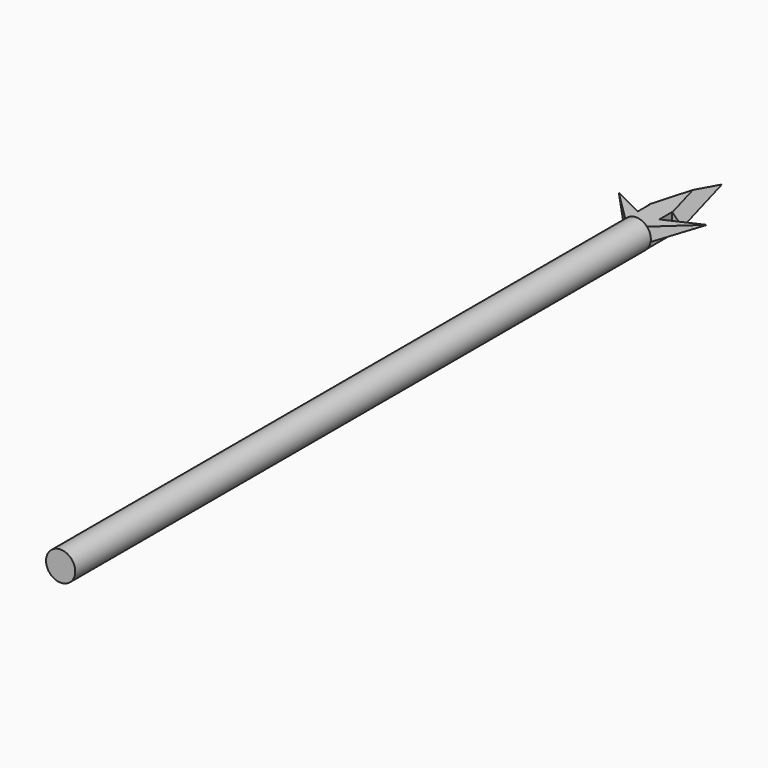
from build123d import *

# Parameters (mm, degrees)
F0_R          = 3.81
F1_DEPTH      = 187.71276
F3_DEPTH      = 2.54
F3_DEPTH_BACK = 2.59802
F4_SIZE       = 5.08
F5_T4_DEPTH   = 56.2135595652
F5_T10_DEPTH  = 56.3150595014
F5_T17_DEPTH  = 56.2135595652
F5_T21_DEPTH  = 56.3150595014
F6_T4_DEPTH   = 35.2698827679
F6_T9_DEPTH   = 36.002021323


# Not quite as in the source:
# - a fillet or chamfer that OpenCascade refuses, or shapes differently, is made with other operations: its cross-section is extruded or revolved along the edge and cut away or added


with BuildPart() as f1:
    # F0 (on Front) → F1 (new body)
    with BuildSketch(Plane.XZ):
        Circle(F0_R)
    extrude(amount=-F1_DEPTH)


with BuildPart() as f3:
    # F2 (on Top) → F3 (new body, two sides)
    with BuildSketch(Plane.XY) as f3_sk:
        Polygon((-2.8854149859, 191.8134321757), (-2.8854149859, 187.7436647788), (2.7261148207, 187.7214848121), (2.7261148207, 191.8280913989), (2.7261148207, 195.9346979856), (8.1146247685, 195.9346979856), (0, 224.9049544334), (-8.3053142529, 195.8831995726), (-2.8854149859, 195.8831995726), align=None)
        Polygon((-11.071106419, 195.8831995726), (-2.8854149859, 187.7436647788), (-2.8854149859, 191.8134321757), align=None)
        Polygon((2.7261148207, 191.8280913989), (2.7261148207, 187.7214848121), (11.7052067071, 195.9349513054), align=None)
    extrude(amount=F3_DEPTH)
    extrude(f3_sk.sketch, amount=-F3_DEPTH_BACK)

    # F4
    f4_edges = [f3.edges().sort_by_distance(p)[0] for p in [
        (4.057312, 210.419826, -2.59802),
        (-4.152657, 210.394077, -2.59802),
    ]]
    chamfer(f4_edges, length=F4_SIZE)

    # F5: chamfer of 5.08 on 2 edges, made by hand


with BuildPart() as f5_tool2:
    # F5_s3 → F5_t4 (new body)
    with BuildSketch(Plane(origin=(-46.7750694582, 166.9930275555, 0), x_dir=(0, 0, 1), z_dir=(-0.2697209417, 0.9629385305, 0))):
        with BuildLine():
            Line((-2.6836840979, 60.8052602015), (2.6836840979, 55.4378920056))
            Line((2.6836840979, 55.4378920056), (2.7852840979, 55.4378920056))
            ThreePointArc((2.7852840979, 55.4378920056), (2.6416, 58.0497340546), (2.6416, 60.6615761036))
            Line((2.6416, 60.6615761036), (2.54, 60.7631761036))
            ThreePointArc((2.54, 60.7631761036), (-0.071842049, 60.7631761036), (-2.6836840979, 60.9068602015))
            Line((-2.6836840979, 60.9068602015), (-2.6836840979, 60.8052602015))
        make_face()
    extrude(amount=F5_T4_DEPTH)

    split(bisect_by=Plane.XZ.offset(-195.9346979856), keep=Keep.BOTTOM)

    split(bisect_by=Plane(origin=(-59.4902437107, 17.0246482808, 0), x_dir=(0, 0, 1), z_dir=(0.9614067403, -0.275131023, 0)), keep=Keep.TOP)


with BuildPart() as f3_1:
    add(f3.part)

    # F5_t1: cut F5_tool2
    add(f5_tool2.part, mode=Mode.SUBTRACT)


with BuildPart() as f5_tool8:
    # F5_s9 → F5_t10 (new body)
    with BuildSketch(Plane(origin=(63.0845965483, 220.4402676135, 0), x_dir=(0, 0, 1), z_dir=(-0.275131023, -0.9614067403, 0))):
        with BuildLine():
            Line((2.6836840979, 56.6546460819), (-2.6836840979, 62.0220142778))
            Line((-2.6836840979, 62.0220142778), (-2.6836840979, 62.1236142778))
            ThreePointArc((-2.6836840979, 62.1236142778), (-0.071842049, 61.9799301798), (2.54, 61.9799301798))
            Line((2.54, 61.9799301798), (2.6416, 61.8783301798))
            ThreePointArc((2.6416, 61.8783301798), (2.6416, 59.2664881309), (2.7852840979, 56.6546460819))
            Line((2.7852840979, 56.6546460819), (2.6836840979, 56.6546460819))
        make_face()
    extrude(amount=F5_T10_DEPTH)

    split(bisect_by=Plane.XZ.offset(-195.8831995726), keep=Keep.BOTTOM)

    split(bisect_by=Plane(origin=(58.4133689537, 16.3616974319, 0), x_dir=(0, 0, 1), z_dir=(-0.9629385305, -0.2697209417, 0)), keep=Keep.TOP)


with BuildPart() as f3_2:
    add(f3_1.part)

    # F5_t7: cut F5_tool8
    add(f5_tool8.part, mode=Mode.SUBTRACT)


with BuildPart() as f5_tool15:
    # F5_s16 → F5_t17 (new body)
    with BuildSketch(Plane(origin=(-46.7750694582, 166.9930275555, 0), x_dir=(0, 0, 1), z_dir=(-0.2697209417, 0.9629385305, 0))):
        with BuildLine():
            Line((-2.6836840979, 60.8052602015), (2.6836840979, 55.4378920056))
            Line((2.6836840979, 55.4378920056), (2.7852840979, 55.4378920056))
            ThreePointArc((2.7852840979, 55.4378920056), (2.6416, 58.0497340546), (2.6416, 60.6615761036))
            Line((2.6416, 60.6615761036), (2.54, 60.7631761036))
            ThreePointArc((2.54, 60.7631761036), (-0.071842049, 60.7631761036), (-2.6836840979, 60.9068602015))
            Line((-2.6836840979, 60.9068602015), (-2.6836840979, 60.8052602015))
        make_face()
    extrude(amount=F5_T17_DEPTH)

    split(bisect_by=Plane(origin=(-59.4902437107, 17.0246482808, 0), x_dir=(0, 0, 1), z_dir=(-0.9614067403, 0.275131023, 0)), keep=Keep.TOP)


with BuildPart() as f5_tool19:
    # F5_s20 → F5_t21 (new body)
    with BuildSketch(Plane(origin=(63.0845965483, 220.4402676135, 0), x_dir=(0, 0, 1), z_dir=(-0.275131023, -0.9614067403, 0))):
        with BuildLine():
            Line((2.6836840979, 56.6546460819), (-2.6836840979, 62.0220142778))
            Line((-2.6836840979, 62.0220142778), (-2.6836840979, 62.1236142778))
            ThreePointArc((-2.6836840979, 62.1236142778), (-0.071842049, 61.9799301798), (2.54, 61.9799301798))
            Line((2.54, 61.9799301798), (2.6416, 61.8783301798))
            ThreePointArc((2.6416, 61.8783301798), (2.6416, 59.2664881309), (2.7852840979, 56.6546460819))
            Line((2.7852840979, 56.6546460819), (2.6836840979, 56.6546460819))
        make_face()
    extrude(amount=F5_T21_DEPTH)

    split(bisect_by=Plane(origin=(58.4133689537, 16.3616974319, 0), x_dir=(0, 0, 1), z_dir=(0.9629385305, 0.2697209417, 0)), keep=Keep.TOP)


with BuildPart() as f5_tool15_1:
    add(f5_tool15.part)

    # F5_t23: intersect F5_tool19
    add(f5_tool19.part, mode=Mode.INTERSECT)


with BuildPart() as f3_3:
    add(f3_2.part)

    # F5_t13: cut F5_tool15
    add(f5_tool15_1.part, mode=Mode.SUBTRACT)

    # F6: chamfer of 5.08 on 2 edges, made by hand


with BuildPart() as f6_tool2:
    # F6_s3 → F6_t4 (new body)
    with BuildSketch(Plane(origin=(-67.0801622098, 33.3509587273, 0), x_dir=(0, 0, 1), z_dir=(-0.895434728, 0.4451928211, 0))):
        Polygon((-2.59802, 165.3918424207), (2.48198, 170.4718424207), (-2.59802, 170.4718424207), align=None)
    extrude(amount=F6_T4_DEPTH)

    split(bisect_by=Plane.YZ.offset(-2.8854149859), keep=Keep.BOTTOM)


with BuildPart() as f3_4:
    add(f3_3.part)

    # F6_t1: cut F6_tool2
    add(f6_tool2.part, mode=Mode.SUBTRACT)


with BuildPart() as f6_tool7:
    # F6_s8 → F6_t9 (new body)
    with BuildSketch(Plane(origin=(95.6732562057, 43.7590643917, 0), x_dir=(0, 0, 1), z_dir=(-0.9093928041, -0.4159383703, 0))):
        Polygon((-2.59802, 168.2331901799), (2.48198, 173.3131901799), (-2.59802, 173.3131901799), align=None)
    extrude(amount=F6_T9_DEPTH)

    split(bisect_by=Plane.YZ.offset(2.7261148207), keep=Keep.TOP)


with BuildPart() as f3_5:
    add(f3_4.part)

    # F6_t6: cut F6_tool7
    add(f6_tool7.part, mode=Mode.SUBTRACT)


solid = Compound([f1.part, f3_5.part])
